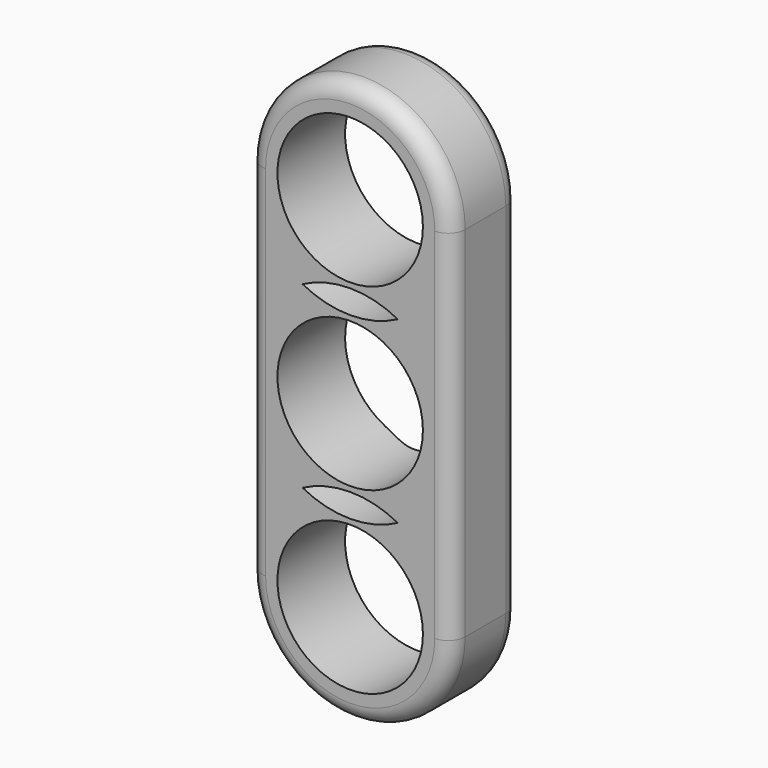
from build123d import *

# Parameters (mm, degrees)
F0_R         = 21.5
F1_DEPTH     = 25
F2_T1_DEPTH  = 106
F2_T4_ANGLE  = 180
F2_T8_ANGLE  = 103.6596556564
F2_S9_R      = 30
F2_T10_DEPTH = 37
F2_T12_ANGLE = 180
F2_T14_ANGLE = 180
F2_T16_ANGLE = 180


# Not quite as in the source:
# - a fillet or chamfer that OpenCascade refuses, or shapes differently, is made with other operations: its cross-section is extruded or revolved along the edge and cut away or added


with BuildPart() as f1:
    # F0 (on Front) → F1 (new body)
    with BuildSketch(Plane.XZ):
        with BuildLine():
            ThreePointArc((14.0623611104, -26.5), (25.7086642332, -15.4617134673), (30, 0))
            ThreePointArc((30, 0), (25.7086642332, 15.4617134673), (14.0623611104, 26.5))
            ThreePointArc((14.0623611104, 26.5), (0, 23), (-14.0623611104, 26.5))
            ThreePointArc((-14.0623611104, 26.5), (-25.7086642332, 15.4617134673), (-30, 0))
            ThreePointArc((-30, 0), (-25.7086642332, -15.4617134673), (-14.0623611104, -26.5))
            ThreePointArc((-14.0623611104, -26.5), (0, -23), (14.0623611104, -26.5))
        make_face()
        Circle(F0_R, mode=Mode.SUBTRACT)
        with BuildLine():
            Line((30, -53), (30, 0))
            ThreePointArc((30, 0), (25.7086642332, -15.4617134673), (14.0623611104, -26.5))
            ThreePointArc((14.0623611104, -26.5), (25.7086642332, -37.5382865327), (30, -53))
        make_face()
        with BuildLine():
            ThreePointArc((14.0623611104, 26.5), (25.7086642332, 15.4617134673), (30, 0))
            Line((30, 0), (30, 53))
            ThreePointArc((30, 53), (25.7086642332, 37.5382865327), (14.0623611104, 26.5))
        make_face()
        with BuildLine():
            ThreePointArc((-14.0623611104, 26.5), (0, 30), (14.0623611104, 26.5))
            ThreePointArc((14.0623611104, 26.5), (25.7086642332, 37.5382865327), (30, 53))
            ThreePointArc((30, 53), (0, 83), (-30, 53))
            ThreePointArc((-30, 53), (-25.7086642332, 37.5382865327), (-14.0623611104, 26.5))
        make_face()
        with Locations((0, 53)):
            Circle(F0_R, mode=Mode.SUBTRACT)
        with BuildLine():
            ThreePointArc((30, -53), (25.7086642332, -37.5382865327), (14.0623611104, -26.5))
            ThreePointArc((14.0623611104, -26.5), (0, -30), (-14.0623611104, -26.5))
            ThreePointArc((-14.0623611104, -26.5), (-25.7086642332, -37.5382865327), (-30, -53))
            ThreePointArc((-30, -53), (0, -83), (30, -53))
        make_face()
        with Locations((0, -53)):
            Circle(F0_R, mode=Mode.SUBTRACT)
        with BuildLine():
            ThreePointArc((-30, 0), (-25.7086642332, 15.4617134673), (-14.0623611104, 26.5))
            ThreePointArc((-14.0623611104, 26.5), (-25.7086642332, 37.5382865327), (-30, 53))
            Line((-30, 53), (-30, 0))
        make_face()
        with BuildLine():
            ThreePointArc((-30, -53), (-25.7086642332, -37.5382865327), (-14.0623611104, -26.5))
            ThreePointArc((-14.0623611104, -26.5), (-25.7086642332, -15.4617134673), (-30, 0))
            Line((-30, 0), (-30, -53))
        make_face()
    extrude(amount=F1_DEPTH)

    # F2: fillet of radius 5 on 3 edges, made by hand

    # F2_s2 → F2_t1 (cut)
    with BuildSketch(Plane.XY.offset(-53)):
        with BuildLine():
            ThreePointArc((-30, -20), (-28.5355339059, -23.5355339059), (-25, -25))
            Line((-25, -25), (-25, -25.1))
            Line((-25, -25.1), (-30.1, -25.1))
            Line((-30.1, -25.1), (-30.1, -20))
            Line((-30.1, -20), (-30, -20))
        make_face()
        with BuildLine():
            ThreePointArc((-30, -5), (-28.5355339059, -1.4644660941), (-25, 0))
            Line((-25, 0), (-25, 0.1))
            Line((-25, 0.1), (-30.1, 0.1))
            Line((-30.1, 0.1), (-30.1, -5))
            Line((-30.1, -5), (-30, -5))
        make_face()
        with BuildLine():
            ThreePointArc((30, -5), (28.5355339059, -1.4644660941), (25, 0))
            Line((25, 0), (25, 0.1))
            Line((25, 0.1), (30.1, 0.1))
            Line((30.1, 0.1), (30.1, -5))
            Line((30.1, -5), (30, -5))
        make_face()
        with BuildLine():
            ThreePointArc((30, -20), (28.5355339059, -23.5355339059), (25, -25))
            Line((25, -25), (25, -25.1))
            Line((25, -25.1), (30.1, -25.1))
            Line((30.1, -25.1), (30.1, -20))
            Line((30.1, -20), (30, -20))
        make_face()
    extrude(amount=F2_T1_DEPTH, mode=Mode.SUBTRACT)

    # F2_s3 → F2_t4 (revolve, cut)
    with BuildSketch(Plane.XY.offset(-53)):
        with BuildLine():
            ThreePointArc((-30, -5), (-28.5355339059, -1.4644660941), (-25, 0))
            Line((-25, 0), (-25, 0.1))
            Line((-25, 0.1), (-30.1, 0.1))
            Line((-30.1, 0.1), (-30.1, -5))
            Line((-30.1, -5), (-30, -5))
        make_face()
    revolve(axis=Axis((0, 0, -53), (0, -1, 0)), revolution_arc=F2_T4_ANGLE, mode=Mode.SUBTRACT)


with BuildPart() as f2_tool6:
    # F2_s7 → F2_t8 (revolve)
    with BuildSketch(Plane(origin=(-25.7504646383, 0, -32.7580804495), x_dir=(0, 1, 0), z_dir=(-0.6179991993, 0, -0.7861787263))):
        with BuildLine():
            ThreePointArc((-5, 2.7539575651), (-1.4644660941, 1.289491471), (0, -2.2460424349))
            Line((0, -2.2460424349), (0.1, -2.2460424349))
            Line((0.1, -2.2460424349), (0.1, 2.8539575651))
            Line((0.1, 2.8539575651), (-5, 2.8539575651))
            Line((-5, 2.8539575651), (-5, 2.7539575651))
        make_face()
    revolve(axis=Axis((0, 0, -53), (0, 1, 0)), revolution_arc=F2_T8_ANGLE)

    # F2_s9 → F2_t10 (intersect, symmetric)
    with BuildSketch(Plane.XZ.offset(4.2)):
        Circle(F2_S9_R)
    extrude(amount=F2_T10_DEPTH, both=True, mode=Mode.INTERSECT)


with BuildPart() as f1_1:
    add(f1.part)

    # F2_t5: cut F2_tool6
    add(f2_tool6.part, mode=Mode.SUBTRACT)

    # F2_s11 → F2_t12 (revolve, cut)
    with BuildSketch(Plane.XY.offset(53)):
        with BuildLine():
            ThreePointArc((30, -5), (28.5355339059, -1.4644660941), (25, 0))
            Line((25, 0), (25, 0.1))
            Line((25, 0.1), (30.1, 0.1))
            Line((30.1, 0.1), (30.1, -5))
            Line((30.1, -5), (30, -5))
        make_face()
    revolve(axis=Axis((0, 0, 53), (0, -1, 0)), revolution_arc=F2_T12_ANGLE, mode=Mode.SUBTRACT)

    # F2_s13 → F2_t14 (revolve, cut)
    with BuildSketch(Plane.XY.offset(53)):
        with BuildLine():
            ThreePointArc((30, -20), (28.5355339059, -23.5355339059), (25, -25))
            Line((25, -25), (25, -25.1))
            Line((25, -25.1), (30.1, -25.1))
            Line((30.1, -25.1), (30.1, -20))
            Line((30.1, -20), (30, -20))
        make_face()
    revolve(axis=Axis((0, -25, 53), (0, -1, 0)), revolution_arc=F2_T14_ANGLE, mode=Mode.SUBTRACT)

    # F2_s15 → F2_t16 (revolve, cut)
    with BuildSketch(Plane.XY.offset(-53)):
        with BuildLine():
            ThreePointArc((-30, -20), (-28.5355339059, -23.5355339059), (-25, -25))
            Line((-25, -25), (-25, -25.1))
            Line((-25, -25.1), (-30.1, -25.1))
            Line((-30.1, -25.1), (-30.1, -20))
            Line((-30.1, -20), (-30, -20))
        make_face()
    revolve(axis=Axis((0, -25, -53), (0, -1, 0)), revolution_arc=F2_T16_ANGLE, mode=Mode.SUBTRACT)


solid = f1_1.part
